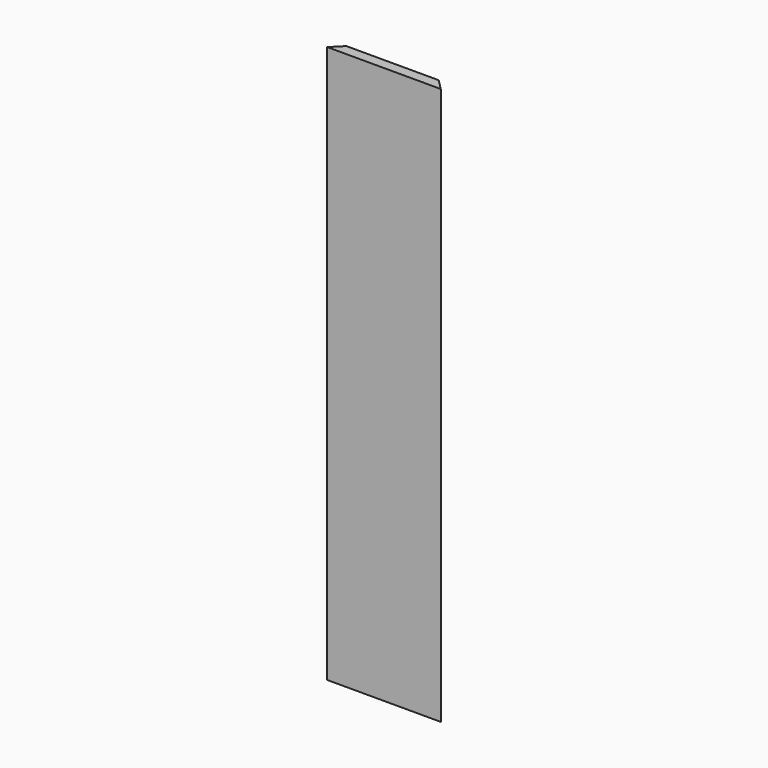
from build123d import *

# Parameters (mm, degrees)
F0_W     = 203.2
F0_H     = 996.95
F1_DEPTH = 19.05
F2_SIZE2 = 19.04999
F2_SIZE  = 19.04999


# Not quite as in the source:
# - a fillet or chamfer is up to 0.001 mm smaller than in the source, because OpenCascade refuses the exact size


with BuildPart() as f1:
    # F0 (on Front) → F1 (new body)
    with BuildSketch(Plane.XZ):
        with Locations((0, -22.3263513706)):
            Rectangle(F0_W, F0_H)
    extrude(amount=F1_DEPTH)

    # F2 (size 19.05 and 19.05 in the source; OpenCascade refuses exactly that, so slightly less here)
    f2_edges = [f1.edges().sort_by_distance(p)[0] for p in [
        (101.6, 0, -22.326351),
        (-101.6, 0, -22.326351),
    ]]
    chamfer(f2_edges, length=F2_SIZE, length2=F2_SIZE2)


solid = f1.part
